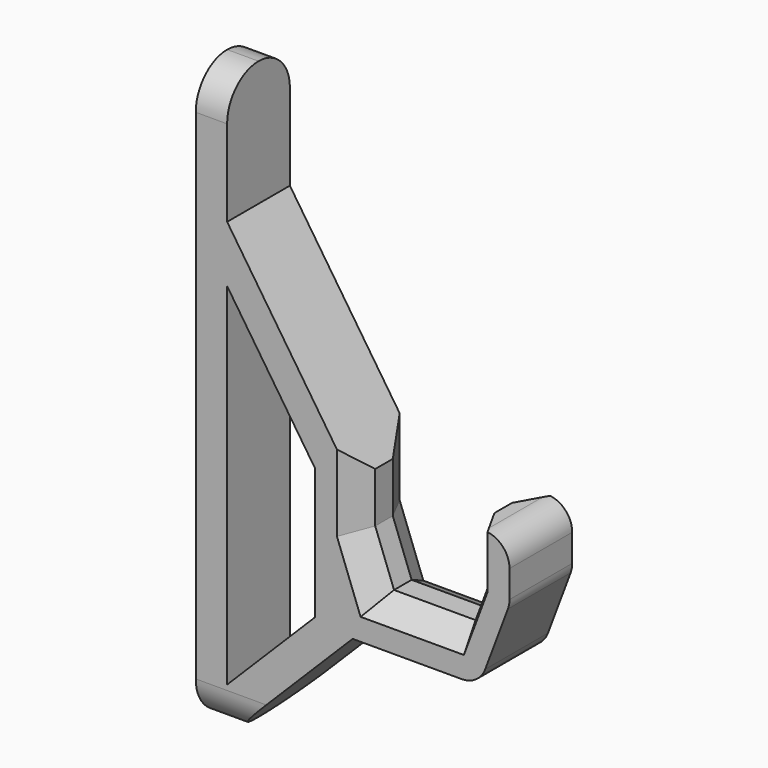
from build123d import *

# Parameters (mm, degrees)
F1_DEPTH = 25
F2_SIZE2 = 5
F2_SIZE  = 9
F3_SIZE2 = 9
F3_SIZE  = 5
F4_R     = 8
F5_R     = 12.49999
F6_SIZE2 = 39.99999
F6_SIZE  = 59.99999
F7_SIZE  = 39.99999
F9_DEPTH = 25.001


# Not quite as in the source:
# - a fillet or chamfer is up to 0.001 mm smaller than in the source, because OpenCascade refuses the exact size


with BuildPart() as f1:
    # F0 (on Front) → F1 (new body)
    with BuildSketch(Plane.XZ):
        Polygon((0, -16), (0, 0), (-40, 0), (-40, 100), (-50, 100), (-50, -84), (-40, -84), (-40, -44), (40.316005618, -44), (50, -18.1760149813), (50, 0), (38, 0), (38, -16), (32, -32), (6, -32), align=None)
    extrude(amount=F1_DEPTH)

    # F2
    f2_edges = [f1.edges().sort_by_distance(p)[0] for p in [
        (19, -25, -32),
        (3, -25, -24),
        (0, -25, -8),
        (35, -25, -24),
        (38, -25, -8),
    ]]
    chamfer(f2_edges, length=F2_SIZE, length2=F2_SIZE2)

    # F3
    f3_edges = [f1.edges().sort_by_distance(p)[0] for p in [
        (19, 0, -32),
        (3, 0, -24),
        (0, 0, -8),
        (35, 0, -24),
        (38, 0, -8),
    ]]
    f3_side = f1.faces().sort_by_distance((-19.786858, 0, -11.21384))[0]
    chamfer(f3_edges, length=F3_SIZE, length2=F3_SIZE2, reference=f3_side)

    # F4
    f4_edges = [f1.edges().sort_by_distance(p)[0] for p in [
        (40.316006, -12.5, -44),
        (50, -12.5, -18.176015),
        (50, -12.5, 0),
    ]]
    fillet(f4_edges, radius=F4_R)

    # F5 (radius 12.5 in the source; OpenCascade refuses exactly that, so slightly less here)
    f5_edges = [f1.edges().sort_by_distance(p)[0] for p in [
        (-45, -25, -84),
        (-45, 0, -84),
        (-45, -25, 100),
        (-45, 0, 100),
    ]]
    fillet(f5_edges, radius=F5_R)

    # F6 (size 60 and 40 in the source; OpenCascade refuses exactly that, so slightly less here)
    f6_edges = [f1.edges().sort_by_distance(p)[0] for p in [
        (-40, -12.5, 0),
    ]]
    f6_side = f1.faces().sort_by_distance((-40, -12.5, 48.698732))[0]
    chamfer(f6_edges, length=F6_SIZE, length2=F6_SIZE2, reference=f6_side)

    # F7 (size 40 in the source; OpenCascade refuses exactly that, so slightly less here)
    f7_edges = [f1.edges().sort_by_distance(p)[0] for p in [
        (-40, -12.5, -44),
    ]]
    chamfer(f7_edges, length=F7_SIZE)

    # F8 (on face) → F9 (cut, through all)
    with BuildSketch(Plane.XZ.offset(25)):
        Polygon((-12, -0.0277563773), (-40, 41.9722436227), (-40, -69.8578643763), (-12, -41.8578643763), align=None)
    extrude(amount=-F9_DEPTH, mode=Mode.SUBTRACT)


solid = f1.part
